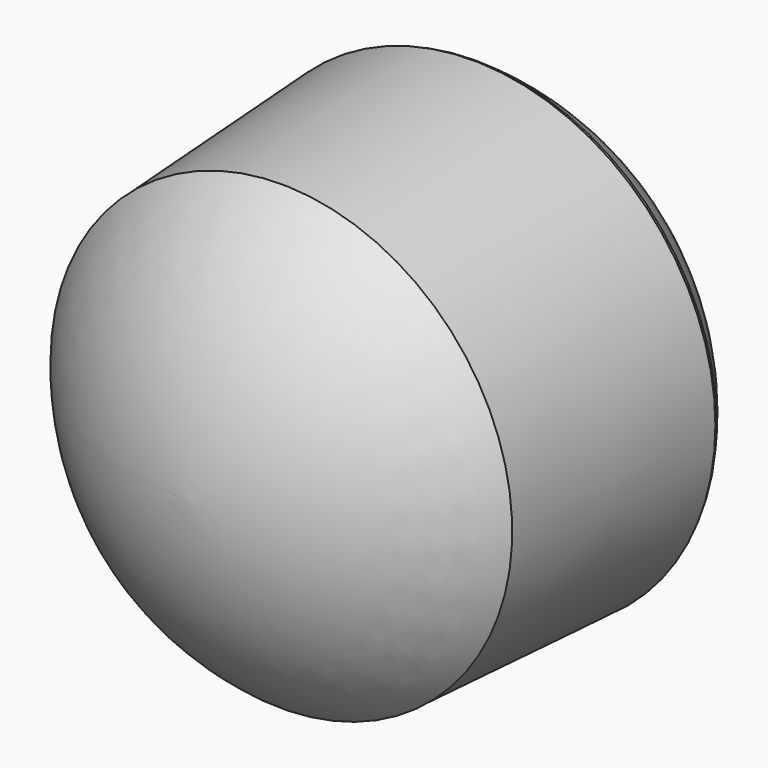
from build123d import *

# Parameters (mm, degrees)
F0_R     = 49.0472883748
F1_DEPTH = 50.8
F1_TAPER = -3
F5_T     = 2.54


# Not quite as in the source:
# - a shell that OpenCascade refuses in one call is made with other operations: the cavity is built on its own and cut out


with BuildPart() as f1:
    # F0 (on Front) → F1 (new body)
    with BuildSketch(Plane.XZ):
        Circle(F0_R)
    extrude(amount=-F1_DEPTH, taper=F1_TAPER)

    # F3 (on Top) → F4 (revolve)
    with BuildSketch(Plane.XY):
        with BuildLine():
            Line((0, -25.114249438), (0, 0))
            Line((0, 0), (-49.1172485054, 0))
            ThreePointArc((-49.1172485054, 0), (-27.4538727535, -18.2195133344), (0, -25.114249438))
        make_face()
    revolve(axis=Axis((0, -12.557124719, 0), (0, -1, 0)))

    # F5: shell of thickness 2.54, made by hand


with BuildPart() as f5_core1:
    # F5_t2: copy of F1
    add(f1.part)

    # the walls: a layer under each face that stays
    f5_faces = [f5_core1.faces().sort_by_distance(p)[0] for p in [
        (42.9775924422, 0, 23.6490455767),
        (27.4538727535, -18.2195133344, 0),
        (-50.3784459686, 25.4, 0),
    ]]
    thicken(f5_faces, amount=-F5_T, mode=Mode.SUBTRACT)

    # F5_s3 → F5_t4 (revolve, cut)
    with BuildSketch(Plane.XY):
        Polygon((49.072653565, 0.0240706667), (49.0472883748, -2.54), (46.3706868566, -2.54), (46.5107693565, 0.1329333289), align=None)
    revolve(axis=Axis((0, 0, 0), (0, 1, 0)), mode=Mode.SUBTRACT)


with BuildPart() as f1_1:
    add(f1.part)

    # what is left inside the walls is the cavity
    f5_cavity = [f5_core1.part.solids().sort_by_distance(p)[0] for p in [
        (-47.394491, 17.480676, 0),
    ]]
    add(f5_cavity, mode=Mode.SUBTRACT)


with BuildPart() as f7:
    # F6 (on Top) → F7 (revolve)
    with BuildSketch(Plane.XY):
        with BuildLine():
            Line((0, 51.0624572635), (0, 74.6690779924))
            ThreePointArc((0, 74.6690779924), (-28.8660068019, 70.3503099814), (-51.2841679156, 51.6600944102))
            Line((-51.2841679156, 51.6600944102), (0, 51.0624572635))
        make_face()
    revolve(axis=Axis((0, -12.3348757625, 0), (0, -1, 0)))


solid = Compound([f1_1.part, f7.part])
